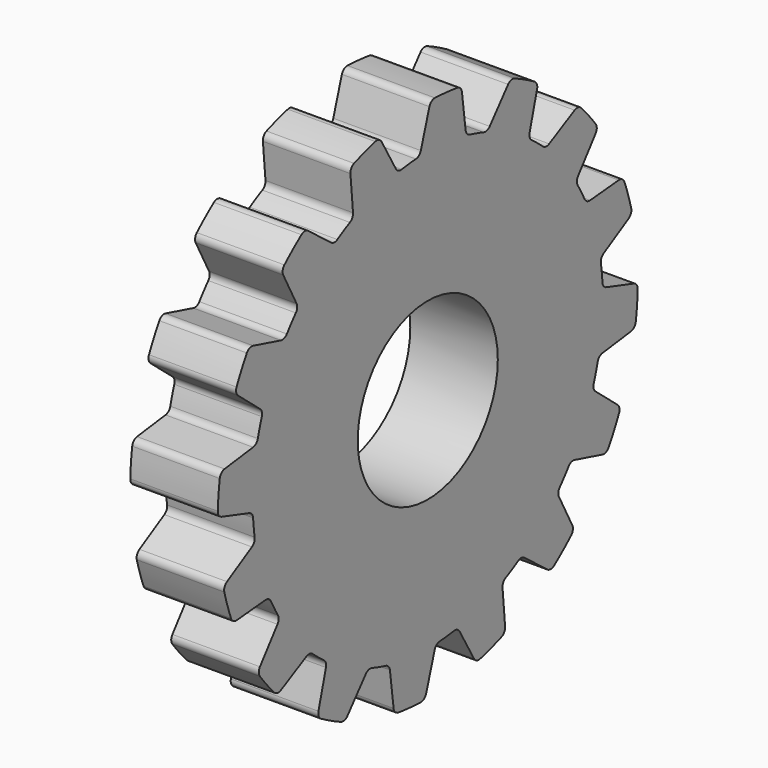
from build123d import *

# Parameters (mm, degrees)
F0_R            = 19.05
F1_DEPTH        = 3.175
F3_DEPTH        = 6.35
F3_COPIES_COUNT = 16
F4_R            = 0.508
F5_R            = 6.35
F6_DEPTH        = 6.35


# Not quite as in the source:
# - a pattern or mirror of a feature is missing from the dataset's text; its kind, count and spacing are read off the source's solid


with BuildPart() as f1:
    # F0 (on Right) → F1 (new body, symmetric)
    with BuildSketch(Plane.YZ):
        Circle(F0_R)
    extrude(amount=F1_DEPTH, both=True)

    # F2 (on face) → F3 (cut, through all)
    with BuildSketch(Plane.YZ.offset(3.175)):
        with BuildLine():
            ThreePointArc((7.5322043505, 17.4976683482), (5.7520331342, 19.7340330411), (3.0490465261, 18.8044094638))
            Line((3.0490465261, 18.8044094638), (3.4766055202, 15.489636505))
            ThreePointArc((3.4766055202, 15.489636505), (4.4423475568, 15.2407733788), (5.3905576771, 14.931761883))
            Line((5.3905576771, 14.931761883), (7.5322043505, 17.4976683482))
        make_face()
    f3 = extrude(amount=-F3_DEPTH, mode=Mode.SUBTRACT)

    # F3_copies: F3 ×16 about axis
    f3_copies_axis = Axis((0, 0, 0), (1, 0, 0))
    for i in range(1, F3_COPIES_COUNT):
        add(f3.rotate(f3_copies_axis, i * 360 / F3_COPIES_COUNT), mode=Mode.SUBTRACT)

    # F4
    f4_edges = [f1.edges().sort_by_distance(p)[0] for p in [
        (0, 3.476606, 15.489637),
        (0, 5.390558, 14.931762),
        (0, 3.049047, 18.804409),
        (0, 7.532204, 17.497668),
        (0, 10.013088, 16.206189),
        (0, 9.139592, 12.980119),
        (0, 10.694364, 11.732272),
        (0, 13.654917, 13.283288),
        (0, 15.452727, 11.140724),
        (0, 13.411158, 8.494496),
        (0, 14.37005, 6.74665),
        (0, 17.698793, 7.046647),
        (0, 18.539829, 4.379184),
        (0, 15.640997, 2.715663),
        (0, 15.858026, 0.733912),
        (0, 19.048187, -0.262782),
        (0, 18.804409, -3.049047),
        (0, 15.489637, -3.476606),
        (0, 14.931762, -5.390558),
        (0, 17.497668, -7.532204),
        (0, 16.206189, -10.013088),
        (0, 12.980119, -9.139592),
        (0, 11.732272, -10.694364),
        (0, 13.283288, -13.654917),
        (0, 11.140724, -15.452727),
        (0, 8.494496, -13.411158),
        (0, 6.74665, -14.37005),
        (0, 7.046647, -17.698793),
        (0, 4.379184, -18.539829),
        (0, 2.715663, -15.640997),
        (0, 0.733912, -15.858026),
        (0, -0.262782, -19.048187),
        (0, -3.049047, -18.804409),
        (0, -3.476606, -15.489637),
        (0, -5.390558, -14.931762),
        (0, -7.532204, -17.497668),
        (0, -10.013088, -16.206189),
        (0, -9.139592, -12.980119),
        (0, -10.694364, -11.732272),
        (0, -13.654917, -13.283288),
        (0, -15.452727, -11.140724),
        (0, -13.411158, -8.494496),
        (0, -14.37005, -6.74665),
        (0, -17.698793, -7.046647),
        (0, -18.539829, -4.379184),
        (0, -15.640997, -2.715663),
        (0, -15.858026, -0.733912),
        (0, -19.048187, 0.262782),
        (0, -18.804409, 3.049047),
        (0, -15.489637, 3.476606),
        (0, -14.931762, 5.390558),
        (0, -17.497668, 7.532204),
        (0, -16.206189, 10.013088),
        (0, -12.980119, 9.139592),
        (0, -11.732272, 10.694364),
        (0, -13.283288, 13.654917),
        (0, -11.140724, 15.452727),
        (0, -8.494496, 13.411158),
        (0, -6.74665, 14.37005),
        (0, -7.046647, 17.698793),
        (0, -4.379184, 18.539829),
        (0, -2.715663, 15.640997),
        (0, -0.733912, 15.858026),
        (0, 0.262782, 19.048187),
    ]]
    fillet(f4_edges, radius=F4_R)

    # F5 (on face) → F6 (cut, through all)
    with BuildSketch(Plane.YZ.offset(3.175)):
        Circle(F5_R)
    extrude(amount=-F6_DEPTH, mode=Mode.SUBTRACT)


solid = f1.part
